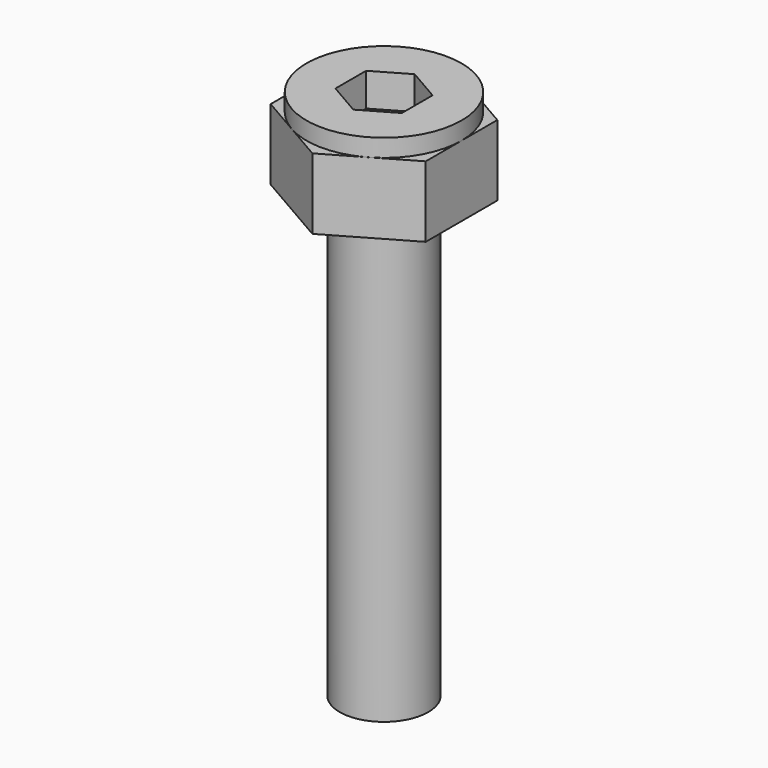
from build123d import *

# Parameters (mm, degrees)
F0_R     = 3.5
F1_DEPTH = 4
F3_DEPTH = 1.5
F4_R     = 2
F5_DEPTH = 20
F7_DEPTH = 3.2
F8_R     = 2
F9_DEPTH = 25


with BuildPart() as f1:
    # F0 (on Top) → F1 (new body)
    with BuildSketch(Plane.XY):
        Circle(F0_R)
    extrude(amount=F1_DEPTH)

    # F2 (on face) → F3 (cut)
    with BuildSketch(Plane.XY.offset(4)):
        Polygon((1.5, 0.8660254038), (0, 1.7320508076), (-1.5, 0.8660254038), (-1.5, -0.8660254038), (0, -1.7320508076), (1.5, -0.8660254038), align=None)
    extrude(amount=-F3_DEPTH, mode=Mode.SUBTRACT)

    # F4 (on face) → F5 (join)
    with BuildSketch(Plane(origin=(0, 0, 0), x_dir=(1, 0, 0), z_dir=(0, 0, -1))):
        Circle(F4_R)
    extrude(amount=F5_DEPTH)


with BuildPart() as f7:
    # F6 (on Top) → F7 (new body)
    with BuildSketch(Plane.XY):
        Polygon((3.5, 2.0207259422), (0, 4.0414518843), (-3.5, 2.0207259422), (-3.5, -2.0207259422), (0, -4.0414518843), (3.5, -2.0207259422), align=None)
    extrude(amount=F7_DEPTH)

    # F8 (on face) → F9 (cut)
    with BuildSketch(Plane.XY.offset(3.2)):
        Circle(F8_R)
    extrude(amount=-F9_DEPTH, mode=Mode.SUBTRACT)


solid = Compound([f1.part, f7.part])
